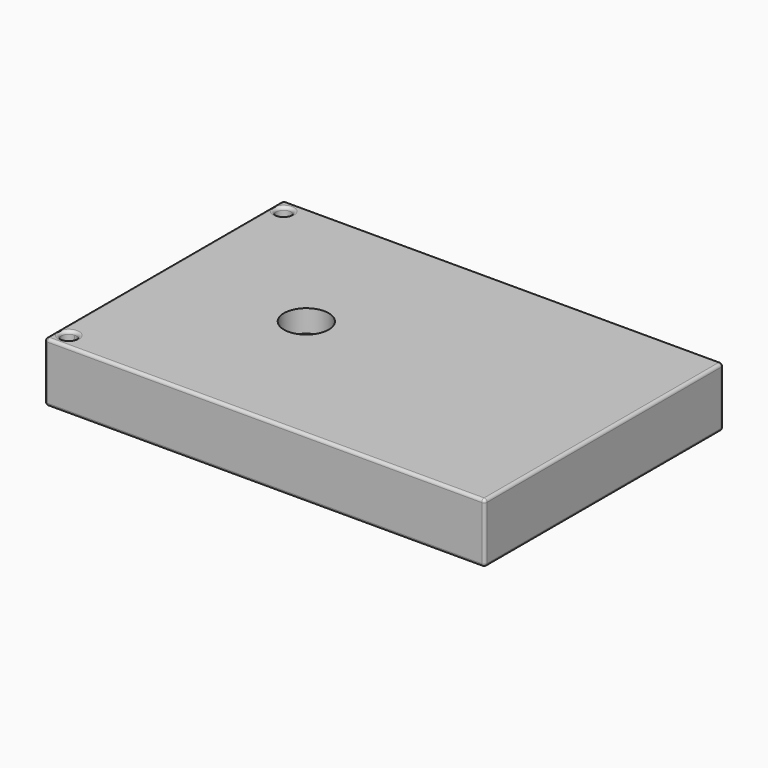
from build123d import *

# Parameters (mm, degrees)
F0_W         = 749.3
F0_H         = 508
F1_DEPTH     = 101.6
F3_DEPTH     = 30.48
F4_T1_DEPTH  = 739.1380686292
F4_T3_DEPTH  = 497.8380686292
F4_T5_DEPTH  = 91.4380686292
F4_S9_W      = 5.5895022539
F4_S9_H      = 5.5895022539
F4_T10_DEPTH = 5.589502254
F4_S15_W     = 5.5895022539
F4_S15_H     = 5.5895022539
F4_T16_DEPTH = 5.589502254
F4_S21_W     = 5.5895022539
F4_S21_H     = 5.5895022539
F4_T22_DEPTH = 5.589502254
F4_S27_W     = 5.5895022539
F4_S27_H     = 5.5895022539
F4_T28_DEPTH = 5.589502254
F4_S33_W     = 5.5895022539
F4_S33_H     = 5.5895022539
F4_T34_DEPTH = 5.589502254
F4_S39_W     = 5.5895022539
F4_S39_H     = 5.5895022539
F4_T40_DEPTH = 5.589502254
F4_S45_W     = 5.5895022539
F4_S45_H     = 5.5895022539
F4_T46_DEPTH = 5.589502254
F4_S51_W     = 5.5895022539
F4_S51_H     = 5.5895022539
F4_T52_DEPTH = 5.589502254
F5_R         = 3.175
F6_DEPTH     = 38.1
F7_R         = 38.1
F8_DEPTH     = 38.1


# Not quite as in the source:
# - a fillet or chamfer that OpenCascade refuses, or shapes differently, is made with other operations: its cross-section is extruded or revolved along the edge and cut away or added


with BuildPart() as f1:
    # F0 (on Top) → F1 (new body)
    with BuildSketch(Plane.XY):
        Rectangle(F0_W, F0_H)
    extrude(amount=-F1_DEPTH)

    # F2 (on face) → F3 (cut)
    with BuildSketch(Plane.XY):
        with BuildLine():
            ThreePointArc((-353.6874055862, 215.9), (-344.7071494652, 219.6197438789), (-340.9874055862, 228.6))
            ThreePointArc((-340.9874055862, 228.6), (-362.6676617073, 237.5802561211), (-353.6874055862, 215.9))
        make_face()
        with BuildLine():
            ThreePointArc((-340.9874055862, -228.6), (-344.7071494652, -219.6197438789), (-353.6874055862, -215.9))
            ThreePointArc((-353.6874055862, -215.9), (-362.6676617073, -237.5802561211), (-340.9874055862, -228.6))
        make_face()
    extrude(amount=-F3_DEPTH, mode=Mode.SUBTRACT)

    # F4: fillet of radius 5.08 on 14 edges, made by hand

    # F4_s2 → F4_t1 (cut)
    with BuildSketch(Plane.YZ.offset(-369.5690343146)):
        with BuildLine():
            ThreePointArc((-254.0004, -5.0809656854), (-252.5121024484, -1.4878975516), (-248.9190343146, 0.0004))
            Line((-248.9190343146, 0.0004), (-248.9190343146, 0.5085365685))
            ThreePointArc((-248.9190343146, 0.5085365685), (-251.4595171573, 0.5081365685), (-254, 0.5081365685))
            Line((-254, 0.5081365685), (-254.5081365685, 0))
            ThreePointArc((-254.5081365685, 0), (-254.5081365685, -2.5404828427), (-254.5085365685, -5.0809656854))
            Line((-254.5085365685, -5.0809656854), (-254.0004, -5.0809656854))
        make_face()
        with BuildLine():
            ThreePointArc((248.9190343146, 0.0004), (252.5121024484, -1.4878975516), (254.0004, -5.0809656854))
            Line((254.0004, -5.0809656854), (254.5085365685, -5.0809656854))
            ThreePointArc((254.5085365685, -5.0809656854), (254.5081365685, -2.5404828427), (254.5081365685, 0))
            Line((254.5081365685, 0), (254, 0.5081365685))
            ThreePointArc((254, 0.5081365685), (251.4595171573, 0.5081365685), (248.9190343146, 0.5085365685))
            Line((248.9190343146, 0.5085365685), (248.9190343146, 0.0004))
        make_face()
        with BuildLine():
            ThreePointArc((-254.0004, -96.5190343146), (-252.5121024484, -100.1121024484), (-248.9190343146, -101.6004))
            Line((-248.9190343146, -101.6004), (-248.9190343146, -102.1085365685))
            ThreePointArc((-248.9190343146, -102.1085365685), (-251.4595171573, -102.1081365685), (-254, -102.1081365685))
            Line((-254, -102.1081365685), (-254.5081365685, -101.6))
            ThreePointArc((-254.5081365685, -101.6), (-254.5081365685, -99.0595171573), (-254.5085365685, -96.5190343146))
            Line((-254.5085365685, -96.5190343146), (-254.0004, -96.5190343146))
        make_face()
        with BuildLine():
            ThreePointArc((248.9190343146, -101.6004), (252.5121024484, -100.1121024484), (254.0004, -96.5190343146))
            Line((254.0004, -96.5190343146), (254.5085365685, -96.5190343146))
            ThreePointArc((254.5085365685, -96.5190343146), (254.5081365685, -99.0595171573), (254.5081365685, -101.6))
            Line((254.5081365685, -101.6), (254, -102.1081365685))
            ThreePointArc((254, -102.1081365685), (251.4595171573, -102.1081365685), (248.9190343146, -102.1085365685))
            Line((248.9190343146, -102.1085365685), (248.9190343146, -101.6004))
        make_face()
    extrude(amount=F4_T1_DEPTH, mode=Mode.SUBTRACT)

    # F4_s4 → F4_t3 (cut)
    with BuildSketch(Plane.XZ.offset(-248.9190343146)):
        with BuildLine():
            ThreePointArc((-374.6504, -5.0809656854), (-373.1621024484, -1.4878975516), (-369.5690343146, 0.0004))
            Line((-369.5690343146, 0.0004), (-369.5690343146, 0.5085365685))
            ThreePointArc((-369.5690343146, 0.5085365685), (-372.1095171573, 0.5081365685), (-374.65, 0.5081365685))
            Line((-374.65, 0.5081365685), (-375.1581365685, 0))
            ThreePointArc((-375.1581365685, 0), (-375.1581365685, -2.5404828427), (-375.1585365685, -5.0809656854))
            Line((-375.1585365685, -5.0809656854), (-374.6504, -5.0809656854))
        make_face()
        with BuildLine():
            ThreePointArc((374.6504, -5.0809656854), (373.1621024484, -1.4878975516), (369.5690343146, 0.0004))
            Line((369.5690343146, 0.0004), (369.5690343146, 0.5085365685))
            ThreePointArc((369.5690343146, 0.5085365685), (372.1095171573, 0.5081365685), (374.65, 0.5081365685))
            Line((374.65, 0.5081365685), (375.1581365685, 0))
            ThreePointArc((375.1581365685, 0), (375.1581365685, -2.5404828427), (375.1585365685, -5.0809656854))
            Line((375.1585365685, -5.0809656854), (374.6504, -5.0809656854))
        make_face()
        with BuildLine():
            ThreePointArc((374.6504, -96.5190343146), (373.1621024484, -100.1121024484), (369.5690343146, -101.6004))
            Line((369.5690343146, -101.6004), (369.5690343146, -102.1085365685))
            ThreePointArc((369.5690343146, -102.1085365685), (372.1095171573, -102.1081365685), (374.65, -102.1081365685))
            Line((374.65, -102.1081365685), (375.1581365685, -101.6))
            ThreePointArc((375.1581365685, -101.6), (375.1581365685, -99.0595171573), (375.1585365685, -96.5190343146))
            Line((375.1585365685, -96.5190343146), (374.6504, -96.5190343146))
        make_face()
        with BuildLine():
            ThreePointArc((-374.6504, -96.5190343146), (-373.1621024484, -100.1121024484), (-369.5690343146, -101.6004))
            Line((-369.5690343146, -101.6004), (-369.5690343146, -102.1085365685))
            ThreePointArc((-369.5690343146, -102.1085365685), (-372.1095171573, -102.1081365685), (-374.65, -102.1081365685))
            Line((-374.65, -102.1081365685), (-375.1581365685, -101.6))
            ThreePointArc((-375.1581365685, -101.6), (-375.1581365685, -99.0595171573), (-375.1585365685, -96.5190343146))
            Line((-375.1585365685, -96.5190343146), (-374.6504, -96.5190343146))
        make_face()
    extrude(amount=F4_T3_DEPTH, mode=Mode.SUBTRACT)

    # F4_s6 → F4_t5 (cut)
    with BuildSketch(Plane.XY.offset(-96.5190343146)):
        with BuildLine():
            ThreePointArc((-374.6504, 248.9190343146), (-373.1621024484, 252.5121024484), (-369.5690343146, 254.0004))
            Line((-369.5690343146, 254.0004), (-369.5690343146, 254.5085365685))
            ThreePointArc((-369.5690343146, 254.5085365685), (-372.1095171573, 254.5081365685), (-374.65, 254.5081365685))
            Line((-374.65, 254.5081365685), (-375.1581365685, 254))
            ThreePointArc((-375.1581365685, 254), (-375.1581365685, 251.4595171573), (-375.1585365685, 248.9190343146))
            Line((-375.1585365685, 248.9190343146), (-374.6504, 248.9190343146))
        make_face()
        with BuildLine():
            ThreePointArc((-369.5690343146, -254.0004), (-373.1621024484, -252.5121024484), (-374.6504, -248.9190343146))
            Line((-374.6504, -248.9190343146), (-375.1585365685, -248.9190343146))
            ThreePointArc((-375.1585365685, -248.9190343146), (-375.1581365685, -251.4595171573), (-375.1581365685, -254))
            Line((-375.1581365685, -254), (-374.65, -254.5081365685))
            ThreePointArc((-374.65, -254.5081365685), (-372.1095171573, -254.5081365685), (-369.5690343146, -254.5085365685))
            Line((-369.5690343146, -254.5085365685), (-369.5690343146, -254.0004))
        make_face()
        with BuildLine():
            ThreePointArc((369.5690343146, -254.0004), (373.1621024484, -252.5121024484), (374.6504, -248.9190343146))
            Line((374.6504, -248.9190343146), (375.1585365685, -248.9190343146))
            ThreePointArc((375.1585365685, -248.9190343146), (375.1581365685, -251.4595171573), (375.1581365685, -254))
            Line((375.1581365685, -254), (374.65, -254.5081365685))
            ThreePointArc((374.65, -254.5081365685), (372.1095171573, -254.5081365685), (369.5690343146, -254.5085365685))
            Line((369.5690343146, -254.5085365685), (369.5690343146, -254.0004))
        make_face()
        with BuildLine():
            ThreePointArc((374.6504, 248.9190343146), (373.1621024484, 252.5121024484), (369.5690343146, 254.0004))
            Line((369.5690343146, 254.0004), (369.5690343146, 254.5085365685))
            ThreePointArc((369.5690343146, 254.5085365685), (372.1095171573, 254.5081365685), (374.65, 254.5081365685))
            Line((374.65, 254.5081365685), (375.1581365685, 254))
            ThreePointArc((375.1581365685, 254), (375.1581365685, 251.4595171573), (375.1585365685, 248.9190343146))
            Line((375.1585365685, 248.9190343146), (374.6504, 248.9190343146))
        make_face()
    extrude(amount=F4_T5_DEPTH, mode=Mode.SUBTRACT)


with BuildPart() as f4_tool8:
    # F4_s9 → F4_t10 (new body)
    with BuildSketch(Plane.XZ.offset(248.9190343146)):
        with Locations((-372.3637854416, -2.2862145584)):
            Rectangle(F4_S9_W, F4_S9_H)
    extrude(amount=F4_T10_DEPTH)

    # F4_s11 → F4_t12 (revolve, cut)
    with BuildSketch(Plane(origin=(-369.5690343146, -248.9190343146, -5.0809656854), x_dir=(0.7071067812, 0, -0.7071067812), z_dir=(-0.7071067812, 0, -0.7071067812))):
        with BuildLine():
            ThreePointArc((0, -5.0813656854), (5.0813656854, 0), (0, 5.0813656854))
            Line((0, 5.0813656854), (0, -5.0813656854))
        make_face()
    revolve(axis=Axis((-369.5690343146, -248.9190343146, -5.0809656854), (0, -1, 0)), mode=Mode.SUBTRACT)


with BuildPart() as f1_1:
    add(f1.part)

    # F4_t7: cut F4_tool8
    add(f4_tool8.part, mode=Mode.SUBTRACT)


with BuildPart() as f4_tool14:
    # F4_s15 → F4_t16 (new body)
    with BuildSketch(Plane.XZ.offset(248.9190343146)):
        with Locations((372.3637854416, -2.2862145584)):
            Rectangle(F4_S15_W, F4_S15_H)
    extrude(amount=F4_T16_DEPTH)

    # F4_s17 → F4_t18 (revolve, cut)
    with BuildSketch(Plane(origin=(369.5690343146, -248.9190343146, -5.0809656854), x_dir=(-0.7071067812, 0, -0.7071067812), z_dir=(-0.7071067812, 0, 0.7071067812))):
        with BuildLine():
            ThreePointArc((0, -5.0813656854), (5.0813656854, 0), (0, 5.0813656854))
            Line((0, 5.0813656854), (0, -5.0813656854))
        make_face()
    revolve(axis=Axis((369.5690343146, -248.9190343146, -5.0809656854), (0, -1, 0)), mode=Mode.SUBTRACT)


with BuildPart() as f1_2:
    add(f1_1.part)

    # F4_t13: cut F4_tool14
    add(f4_tool14.part, mode=Mode.SUBTRACT)


with BuildPart() as f4_tool20:
    # F4_s21 → F4_t22 (new body)
    with BuildSketch(Plane.YZ.offset(-369.5690343146)):
        with Locations((251.7137854415, -2.2862145584)):
            Rectangle(F4_S21_W, F4_S21_H)
    extrude(amount=-F4_T22_DEPTH)

    # F4_s23 → F4_t24 (revolve, cut)
    with BuildSketch(Plane(origin=(-369.5690343146, 248.9190343146, -5.0809656854), x_dir=(0, -0.7071067812, -0.7071067812), z_dir=(0, 0.7071067812, -0.7071067812))):
        with BuildLine():
            ThreePointArc((0, -5.0813656854), (5.0813656854, 0), (0, 5.0813656854))
            Line((0, 5.0813656854), (0, -5.0813656854))
        make_face()
    revolve(axis=Axis((-369.5690343146, 248.9190343146, -5.0809656854), (-1, 0, 0)), mode=Mode.SUBTRACT)


with BuildPart() as f1_3:
    add(f1_2.part)

    # F4_t19: cut F4_tool20
    add(f4_tool20.part, mode=Mode.SUBTRACT)


with BuildPart() as f4_tool26:
    # F4_s27 → F4_t28 (new body)
    with BuildSketch(Plane.YZ.offset(369.5690343146)):
        with Locations((251.7137854415, -2.2862145584)):
            Rectangle(F4_S27_W, F4_S27_H)
    extrude(amount=F4_T28_DEPTH)

    # F4_s29 → F4_t30 (revolve, cut)
    with BuildSketch(Plane(origin=(369.5690343146, 248.9190343146, -5.0809656854), x_dir=(0, -0.7071067812, -0.7071067812), z_dir=(0, -0.7071067812, 0.7071067812))):
        with BuildLine():
            ThreePointArc((0, -5.0813656854), (5.0813656854, 0), (0, 5.0813656854))
            Line((0, 5.0813656854), (0, -5.0813656854))
        make_face()
    revolve(axis=Axis((369.5690343146, 248.9190343146, -5.0809656854), (1, 0, 0)), mode=Mode.SUBTRACT)


with BuildPart() as f1_4:
    add(f1_3.part)

    # F4_t25: cut F4_tool26
    add(f4_tool26.part, mode=Mode.SUBTRACT)


with BuildPart() as f4_tool32:
    # F4_s33 → F4_t34 (new body)
    with BuildSketch(Plane.XZ.offset(248.9190343146)):
        with Locations((-372.3637854416, -99.3137854416)):
            Rectangle(F4_S33_W, F4_S33_H)
    extrude(amount=F4_T34_DEPTH)

    # F4_s35 → F4_t36 (revolve, cut)
    with BuildSketch(Plane(origin=(-369.5690343146, -248.9190343146, -96.5190343146), x_dir=(0.7071067812, 0, 0.7071067812), z_dir=(0.7071067812, 0, -0.7071067812))):
        with BuildLine():
            ThreePointArc((0, -5.0813656854), (5.0813656854, 0), (0, 5.0813656854))
            Line((0, 5.0813656854), (0, -5.0813656854))
        make_face()
    revolve(axis=Axis((-369.5690343146, -248.9190343146, -96.5190343146), (0, -1, 0)), mode=Mode.SUBTRACT)


with BuildPart() as f1_5:
    add(f1_4.part)

    # F4_t31: cut F4_tool32
    add(f4_tool32.part, mode=Mode.SUBTRACT)


with BuildPart() as f4_tool38:
    # F4_s39 → F4_t40 (new body)
    with BuildSketch(Plane.XZ.offset(248.9190343146)):
        with Locations((372.3637854416, -99.3137854416)):
            Rectangle(F4_S39_W, F4_S39_H)
    extrude(amount=F4_T40_DEPTH)

    # F4_s41 → F4_t42 (revolve, cut)
    with BuildSketch(Plane(origin=(369.5690343146, -248.9190343146, -96.5190343146), x_dir=(-0.7071067812, 0, 0.7071067812), z_dir=(0.7071067812, 0, 0.7071067812))):
        with BuildLine():
            ThreePointArc((0, -5.0813656854), (5.0813656854, 0), (0, 5.0813656854))
            Line((0, 5.0813656854), (0, -5.0813656854))
        make_face()
    revolve(axis=Axis((369.5690343146, -248.9190343146, -96.5190343146), (0, -1, 0)), mode=Mode.SUBTRACT)


with BuildPart() as f1_6:
    add(f1_5.part)

    # F4_t37: cut F4_tool38
    add(f4_tool38.part, mode=Mode.SUBTRACT)


with BuildPart() as f4_tool44:
    # F4_s45 → F4_t46 (new body)
    with BuildSketch(Plane.YZ.offset(369.5690343146)):
        with Locations((251.7137854415, -99.3137854416)):
            Rectangle(F4_S45_W, F4_S45_H)
    extrude(amount=F4_T46_DEPTH)

    # F4_s47 → F4_t48 (revolve, cut)
    with BuildSketch(Plane(origin=(369.5690343146, 248.9190343146, -96.5190343146), x_dir=(0, -0.7071067812, 0.7071067812), z_dir=(0, 0.7071067812, 0.7071067812))):
        with BuildLine():
            ThreePointArc((0, -5.0813656854), (5.0813656854, 0), (0, 5.0813656854))
            Line((0, 5.0813656854), (0, -5.0813656854))
        make_face()
    revolve(axis=Axis((369.5690343146, 248.9190343146, -96.5190343146), (1, 0, 0)), mode=Mode.SUBTRACT)


with BuildPart() as f1_7:
    add(f1_6.part)

    # F4_t43: cut F4_tool44
    add(f4_tool44.part, mode=Mode.SUBTRACT)


with BuildPart() as f4_tool50:
    # F4_s51 → F4_t52 (new body)
    with BuildSketch(Plane.YZ.offset(-369.5690343146)):
        with Locations((251.7137854415, -99.3137854416)):
            Rectangle(F4_S51_W, F4_S51_H)
    extrude(amount=-F4_T52_DEPTH)

    # F4_s53 → F4_t54 (revolve, cut)
    with BuildSketch(Plane(origin=(-369.5690343146, 248.9190343146, -96.5190343146), x_dir=(0, -0.7071067812, 0.7071067812), z_dir=(0, -0.7071067812, -0.7071067812))):
        with BuildLine():
            ThreePointArc((0, -5.0813656854), (5.0813656854, 0), (0, 5.0813656854))
            Line((0, 5.0813656854), (0, -5.0813656854))
        make_face()
    revolve(axis=Axis((-369.5690343146, 248.9190343146, -96.5190343146), (-1, 0, 0)), mode=Mode.SUBTRACT)


with BuildPart() as f1_8:
    add(f1_7.part)

    # F4_t49: cut F4_tool50
    add(f4_tool50.part, mode=Mode.SUBTRACT)

    # F4_s55 → F4_t56 (revolve, cut)
    with BuildSketch(Plane.XZ.offset(228.6)):
        with BuildLine():
            ThreePointArc((-335.9064399008, 0.0004), (-339.4995080347, -1.4878975516), (-340.9878055862, -5.0809656854))
            Line((-340.9878055862, -5.0809656854), (-341.4959421548, -5.0809656854))
            ThreePointArc((-341.4959421548, -5.0809656854), (-341.4955421548, -2.5404828427), (-341.4955421548, 0))
            Line((-341.4955421548, 0), (-340.9874055862, 0.5081365685))
            ThreePointArc((-340.9874055862, 0.5081365685), (-338.4469227435, 0.5081365685), (-335.9064399008, 0.5085365685))
            Line((-335.9064399008, 0.5085365685), (-335.9064399008, 0.0004))
        make_face()
    revolve(axis=Axis((-353.6874055862, -228.6, 0), (0, 0, 1)), mode=Mode.SUBTRACT)

    # F4_s57 → F4_t58 (revolve, cut)
    with BuildSketch(Plane.XZ.offset(-228.6)):
        with BuildLine():
            ThreePointArc((-335.9064399008, 0.0004), (-339.4995080347, -1.4878975516), (-340.9878055862, -5.0809656854))
            Line((-340.9878055862, -5.0809656854), (-341.4959421548, -5.0809656854))
            ThreePointArc((-341.4959421548, -5.0809656854), (-341.4955421548, -2.5404828427), (-341.4955421548, 0))
            Line((-341.4955421548, 0), (-340.9874055862, 0.5081365685))
            ThreePointArc((-340.9874055862, 0.5081365685), (-338.4469227435, 0.5081365685), (-335.9064399008, 0.5085365685))
            Line((-335.9064399008, 0.5085365685), (-335.9064399008, 0.0004))
        make_face()
    revolve(axis=Axis((-353.6874055862, 228.6, 0), (0, 0, 1)), mode=Mode.SUBTRACT)

    # F5 (on face) → F6 (cut)
    with BuildSketch(Plane(origin=(0, 0, -101.6), x_dir=(1, 0, 0), z_dir=(0, 0, -1))):
        with Locations((-341.4336416733, 219.583)):
            Circle(F5_R)
        with Locations((-316.7956416733, 219.583)):
            Circle(F5_R)
        with Locations((-341.4336416733, 165.989)):
            Circle(F5_R)
        with Locations((-316.7956416733, 165.989)):
            Circle(F5_R)
        with Locations((-341.4336416733, -219.583)):
            Circle(F5_R)
        with Locations((-316.7956416733, -219.583)):
            Circle(F5_R)
        with Locations((-316.7956416733, -165.989)):
            Circle(F5_R)
        with Locations((-341.4336416733, -165.989)):
            Circle(F5_R)
        with Locations((341.4336416733, 165.989)):
            Circle(F5_R)
        with Locations((316.7956416733, 165.989)):
            Circle(F5_R)
        with Locations((316.7956416733, 219.583)):
            Circle(F5_R)
        with Locations((341.4336416733, 219.583)):
            Circle(F5_R)
        with Locations((316.7956416733, -165.989)):
            Circle(F5_R)
        with Locations((341.4336416733, -165.989)):
            Circle(F5_R)
        with Locations((316.7956416733, -219.583)):
            Circle(F5_R)
        with Locations((341.4336416733, -219.583)):
            Circle(F5_R)
    extrude(amount=-F6_DEPTH, mode=Mode.SUBTRACT)

    # F7 (on face) → F8 (cut)
    with BuildSketch(Plane.XY):
        with Locations((-132.2444367035, 0)):
            Circle(F7_R)
    extrude(amount=-F8_DEPTH, mode=Mode.SUBTRACT)


solid = f1_8.part
